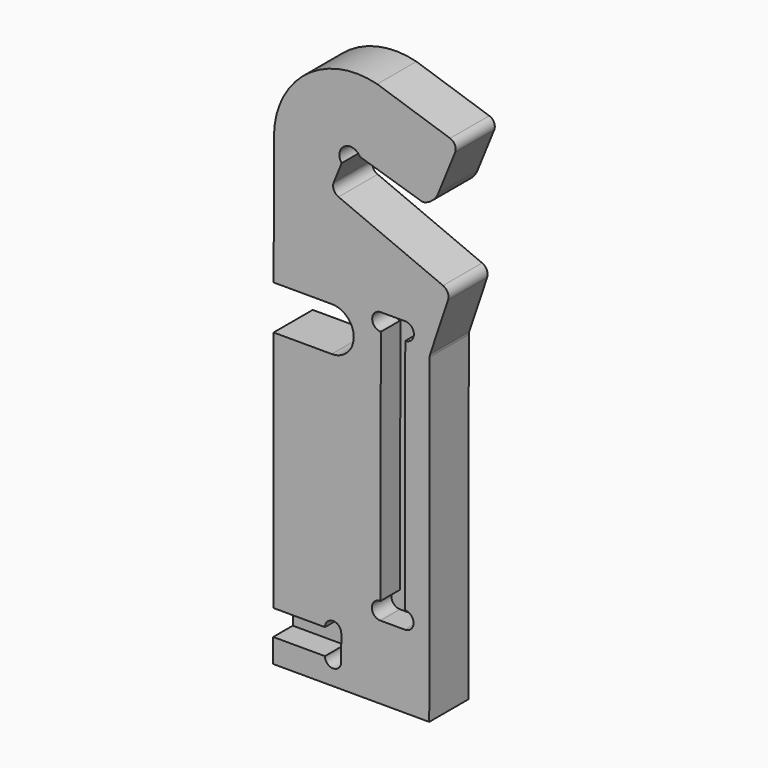
from build123d import *

# Parameters (mm, degrees)
F1_DEPTH = 18
F2_DEPTH = 9


# Not quite as in the source:
# - ends of sketch curves that miss each other by under 0.0002 mm in the source are joined


with BuildPart() as f1:
    # F0 (on Front) → F1 (new body)
    with BuildSketch(Plane.XZ):
        with BuildLine():
            Line((-9.141471, 34.188881), (12.258507, 34.157887))
            ThreePointArc((12.258507, 34.157887), (20.346767, 26.046165), (12.235044, 17.957904))
            Line((12.235044, 17.957904), (-9.164933, 17.988898))
            Line((-9.164933, 17.988898), (-9.294311, -71.341008))
            Line((-9.294311, -71.341008), (9.742649, -71.36858))
            ThreePointArc((9.742649, -71.36858), (12.746991, -68.372928), (15.742643, -71.37727))
            Line((15.742643, -71.37727), (15.729029, -80.77726))
            ThreePointArc((15.729029, -80.77726), (12.724687, -83.772911), (9.729035, -80.76857))
            Line((9.729035, -80.76857), (-9.307925, -80.740999))
            Line((-9.307925, -80.740999), (-9.320635, -89.516989))
            Line((-9.320635, -89.516989), (48.129305, -89.600195))
            Line((48.129305, -89.600195), (48.300632, 28.694563))
            ThreePointArc((48.300632, 28.694563), (48.341618, 29.200469), (48.462079, 29.693531))
            Line((48.462079, 29.693531), (55.053469, 49.381424))
            ThreePointArc((55.053469, 49.381424), (54.931498, 51.787755), (53.20634, 53.469759))
            Line((53.20634, 53.469759), (14.740562, 69.688595))
            ThreePointArc((14.740562, 69.688595), (12.997236, 71.408353), (12.980285, 73.857123))
            Line((12.980285, 73.857123), (15.886835, 81.012644))
            ThreePointArc((15.886835, 81.012644), (16.941219, 86.810977), (22.628344, 85.265342))
            Line((22.628344, 85.265342), (45.010367, 78.329111))
            ThreePointArc((45.010367, 78.329111), (46.013877, 78.196697), (47.004304, 78.405553))
            ThreePointArc((47.004304, 78.405553), (49.689322, 80.161839), (51.468356, 82.83184))
            Line((51.468356, 82.83184), (57.653713, 98.061229))
            ThreePointArc((57.653713, 98.061229), (57.597139, 100.449348), (55.814134, 102.039067))
            Line((55.814134, 102.039067), (28.999419, 110.885722))
            ThreePointArc((28.999419, 110.885722), (2.856816, 105.590311), (-9.035869, 81.714778))
            Line((-9.035869, 81.714778), (-9.141471, 34.188881))
        make_face()
        with BuildLine():
            ThreePointArc((39.177572, -56.266483), (42.347971, -59.446078), (39.168375, -62.616476))
            Line((39.168375, -62.616476), (30.168385, -62.603441))
            ThreePointArc((30.168385, -62.603441), (26.997987, -59.423846), (30.177582, -56.253447))
            Line((30.177582, -56.253447), (30.304019, 31.046461))
            ThreePointArc((30.304019, 31.046461), (27.133621, 34.226056), (30.313216, 37.396454))
            Line((30.313216, 37.396454), (39.313207, 37.383419))
            ThreePointArc((39.313207, 37.383419), (42.483605, 34.203824), (39.30401, 31.033426))
            Line((39.30401, 31.033426), (39.177572, -56.266483))
        make_face(mode=Mode.SUBTRACT)
        with BuildLine():
            Line((30.168385, -62.603441), (39.168375, -62.616476))
            ThreePointArc((39.168375, -62.616476), (42.347971, -59.446078), (39.177572, -56.266483))
            Line((39.177572, -56.266483), (39.30401, 31.033426))
            ThreePointArc((39.30401, 31.033426), (42.483605, 34.203824), (39.313207, 37.383419))
            Line((39.313207, 37.383419), (30.313216, 37.396454))
            ThreePointArc((30.313216, 37.396454), (27.133621, 34.226056), (30.304019, 31.046461))
            Line((30.304019, 31.046461), (30.177582, -56.253448))
            ThreePointArc((30.177582, -56.253448), (26.997987, -59.423846), (30.168385, -62.603441))
        make_face()
        with BuildLine():
            Line((9.742649, -71.36858), (-9.294311, -71.341008))
            Line((-9.294311, -71.341008), (-9.307925, -80.740999))
            Line((-9.307925, -80.740999), (9.729035, -80.76857))
            ThreePointArc((9.729035, -80.76857), (12.724687, -83.772911), (15.729029, -80.77726))
            Line((15.729029, -80.77726), (15.742643, -71.37727))
            ThreePointArc((15.742643, -71.37727), (12.746991, -68.372928), (9.742649, -71.36858))
        make_face()
    extrude(amount=-F1_DEPTH)

    # F0 (on Front) → F2 (cut)
    with BuildSketch(Plane.XZ):
        with BuildLine():
            Line((9.742649, -71.36858), (-9.294311, -71.341008))
            Line((-9.294311, -71.341008), (-9.307925, -80.740999))
            Line((-9.307925, -80.740999), (9.729035, -80.76857))
            ThreePointArc((9.729035, -80.76857), (12.724687, -83.772911), (15.729029, -80.77726))
            Line((15.729029, -80.77726), (15.742643, -71.37727))
            ThreePointArc((15.742643, -71.37727), (12.746991, -68.372928), (9.742649, -71.36858))
        make_face()
        with BuildLine():
            Line((30.168385, -62.603441), (39.168375, -62.616476))
            ThreePointArc((39.168375, -62.616476), (42.347971, -59.446078), (39.177572, -56.266483))
            Line((39.177572, -56.266483), (39.30401, 31.033426))
            ThreePointArc((39.30401, 31.033426), (42.483605, 34.203824), (39.313207, 37.383419))
            Line((39.313207, 37.383419), (30.313216, 37.396454))
            ThreePointArc((30.313216, 37.396454), (27.133621, 34.226056), (30.304019, 31.046461))
            Line((30.304019, 31.046461), (30.177582, -56.253448))
            ThreePointArc((30.177582, -56.253448), (26.997987, -59.423846), (30.168385, -62.603441))
        make_face()
    extrude(amount=-F2_DEPTH, mode=Mode.SUBTRACT)


solid = f1.part
